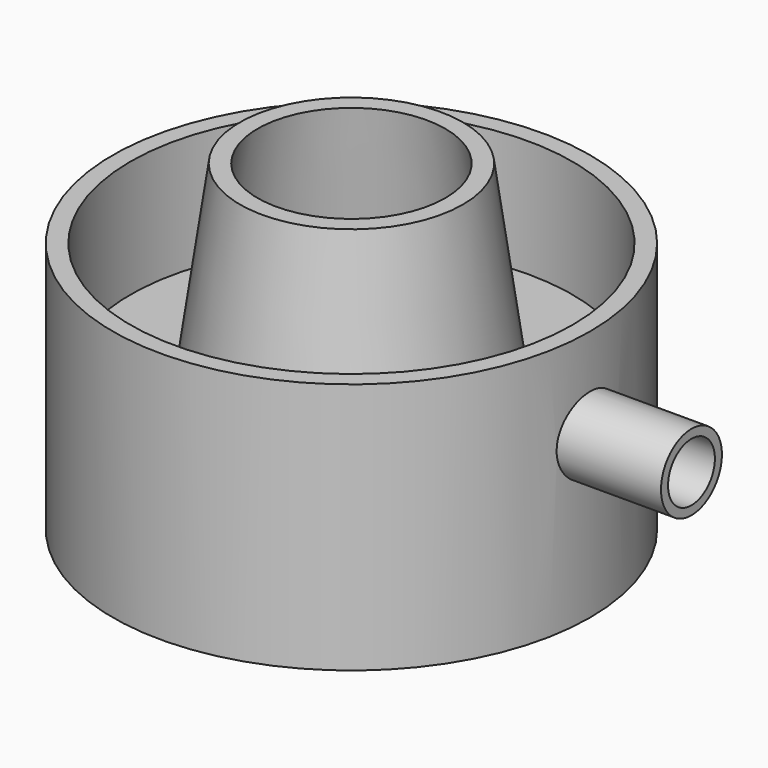
from build123d import *

# Parameters (mm, degrees)
F3_R     = 6.5
F3_R_2   = 5
F4_DEPTH = 20
F5_DEPTH = 14.3


with BuildPart() as f1:
    # F0 (on Front) → F1 (revolve)
    with BuildSketch(Plane.XZ):
        Polygon((-130.0127011951, 91.7292905117), (-133.0127011951, 91.7292905117), (-128.0937719805, 56.7292905117), (-111.2923327753, 56.7292905117), (-111.2923327753, 36.7292905117), (-108.2923327753, 36.7292905117), (-108.2923327753, 79.7292905117), (-111.2923327753, 79.7292905117), (-111.2923327753, 59.7292905117), (-125.5153944847, 59.7292905117), align=None)
    revolve(axis=Axis((-149.0423327753, 0, 54.1304184761), (0, 0, -1)))

    # F3 (on offset) → F4 (join)
    with BuildSketch(Plane.YZ.offset(-111)):
        with Locations((0, 64.2200395022)):
            Circle(F3_R)
        with Locations((0, 64.2200395022)):
            Circle(F3_R_2, mode=Mode.SUBTRACT)
    extrude(amount=F4_DEPTH)

    # F3 (on offset) → F5 (cut, symmetric)
    with BuildSketch(Plane.YZ.offset(-111)):
        with Locations((0, 64.2200395022)):
            Circle(F3_R_2)
    extrude(amount=F5_DEPTH, both=True, mode=Mode.SUBTRACT)


solid = f1.part
